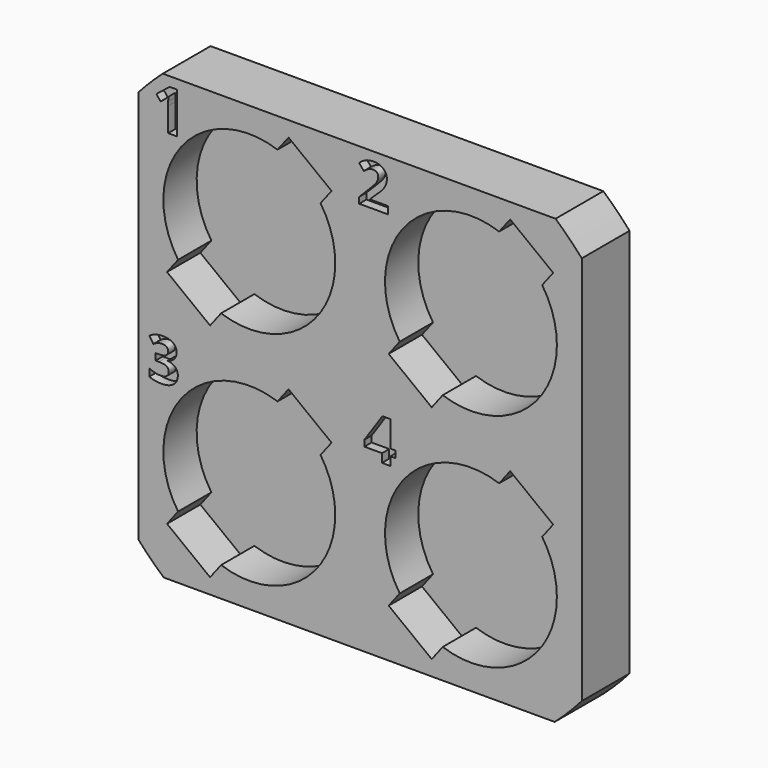
from build123d import *

# Parameters (mm, degrees)
F0_W         = 12.25
F0_H         = 12.25
F1_DEPTH     = 3.3
F3_DEPTH     = 2.3
F8_TEXT_SIZE = 3.1944444444
F9_DEPTH     = 0.5
F11_START    = 0.5
F10_R        = 16.35
F11_DEPTH    = 5
F12_DEPTH    = 0.5


# Not quite as in the source:
# - Text() gives the source's letters only with a copy of the font that has no kerning and outlines rounded to 1/6400 em; it was checked with that copy


with BuildPart() as f1:
    # F0 (on Front) → F1 (new body)
    with BuildSketch(Plane.XZ):
        Rectangle(F0_W, F0_H)
    extrude(amount=-F1_DEPTH)

    # F2 (on Front) → F3 (cut)
    with BuildSketch(Plane.XZ):
        with BuildLine():
            Line((-2.1682334914, -5.2796914413), (-1.5585933765, -4.4870131142))
            ThreePointArc((-1.5585933765, -4.4870131142), (-2.8957905457, -3.7652220539), (-3.936628358, -2.6580927695))
            Line((-3.936628358, -2.6580927695), (-4.5462684729, -3.4507710966))
            Line((-4.5462684729, -3.4507710966), (-2.1682334914, -5.2796914413))
        make_face()
        with BuildLine():
            ThreePointArc((1.5585933765, 4.4870131142), (2.8957905457, 3.7652220539), (3.936628358, 2.6580927695))
            Line((3.936628358, 2.6580927695), (4.5462684729, 3.4507710966))
            Line((4.5462684729, 3.4507710966), (2.1682334914, 5.2796914413))
            Line((2.1682334914, 5.2796914413), (1.5585933765, 4.4870131142))
        make_face()
        with BuildLine():
            ThreePointArc((-1.5585933765, -4.4870131142), (2.7531056519, -3.8707763135), (4.75, 0))
            ThreePointArc((4.75, 0), (4.5421076991, 1.389876847), (3.936628358, 2.6580927695))
            ThreePointArc((3.936628358, 2.6580927695), (2.8957905457, 3.7652220539), (1.5585933765, 4.4870131142))
            ThreePointArc((1.5585933765, 4.4870131142), (-3.7652220539, 2.8957905457), (-3.936628358, -2.6580927695))
            ThreePointArc((-3.936628358, -2.6580927695), (-2.8957905457, -3.7652220539), (-1.5585933765, -4.4870131142))
        make_face()
    extrude(amount=-F3_DEPTH, mode=Mode.SUBTRACT)


with BuildPart() as f4_1:
    # F4: copy of F1
    add(f1.part.moved(Location((-12.25, 0, 0))))


with BuildPart() as f5_1:
    # F5: copy of F1
    add(f1.part.moved(Location((0, 0, 12.25))))


with BuildPart() as f6_1:
    # F6: copy of F1
    add(f1.part.moved(Location((-12.25, 0, 12.25))))


with BuildPart() as f1_1:
    add(f1.part)

    # F7: union F4_1, F5_1, F6_1
    add(f4_1.part)
    add(f5_1.part)
    add(f6_1.part)

    # F8 (on face) → F9 (cut)
    with BuildSketch(Plane.XZ):
        with Locations((-17.575, 15.575)):
            Text('1', F8_TEXT_SIZE, font='Open Sans', font_style=FontStyle.BOLD, text_align=(TextAlign.LEFT, TextAlign.BOTTOM))
        with Locations((-6.3041449653, 15.575)):
            Text('2', F8_TEXT_SIZE, font='Open Sans', font_style=FontStyle.BOLD, text_align=(TextAlign.LEFT, TextAlign.BOTTOM))
        with Locations((-17.9008301879, 3.2952082697)):
            Text('3', F8_TEXT_SIZE, font='Open Sans', font_style=FontStyle.BOLD, text_align=(TextAlign.LEFT, TextAlign.BOTTOM))
        with Locations((-5.9457776095, 3.375)):
            Text('4', F8_TEXT_SIZE, font='Open Sans', font_style=FontStyle.BOLD, text_align=(TextAlign.LEFT, TextAlign.BOTTOM))
    extrude(amount=-F9_DEPTH, mode=Mode.SUBTRACT)

    # F10 (on Front) → F11 (intersect)
    with BuildSketch(Plane.XZ.offset(F11_START)):
        with Locations((-6.1763664708, 6.1472062953)):
            Circle(F10_R)
    extrude(amount=-F11_DEPTH, mode=Mode.INTERSECT)

    # F8 (on face) → F12 (cut)
    with BuildSketch(Plane.XZ):
        with BuildLine():
            Line((-5.4671100748, 4.2220269097), (-4.9180649359, 4.2220269097))
            Line((-4.9180649359, 4.2220269097), (-4.9180649359, 4.6088541667))
            add(Edge.make_bspline(
                [(-4.9180649359, 4.6088541667), (-4.9180649359, 4.7056857639), (-4.9100788248, 4.8896158854)],
                knots=[0, 0, 0, 1, 1, 1], degree=2))
            add(Edge.make_bspline(
                [(-4.9100788248, 4.8896158854), (-4.9020927136, 5.0735460069), (-4.8976005261, 5.1034939236)],
                knots=[0, 0, 0, 1, 1, 1], degree=2))
            Line((-4.8976005261, 5.1034939236), (-4.9100788248, 5.1034939236))
            add(Edge.make_bspline(
                [(-4.9100788248, 5.1034939236), (-4.9679781303, 4.9752170139), (-5.0488375053, 4.8539279514)],
                knots=[0, 0, 0, 1, 1, 1], degree=2))
            Line((-5.0488375053, 4.8539279514), (-5.4671100748, 4.2220269097))
        make_face()
    extrude(amount=-F12_DEPTH, mode=Mode.SUBTRACT)


solid = f1_1.part
